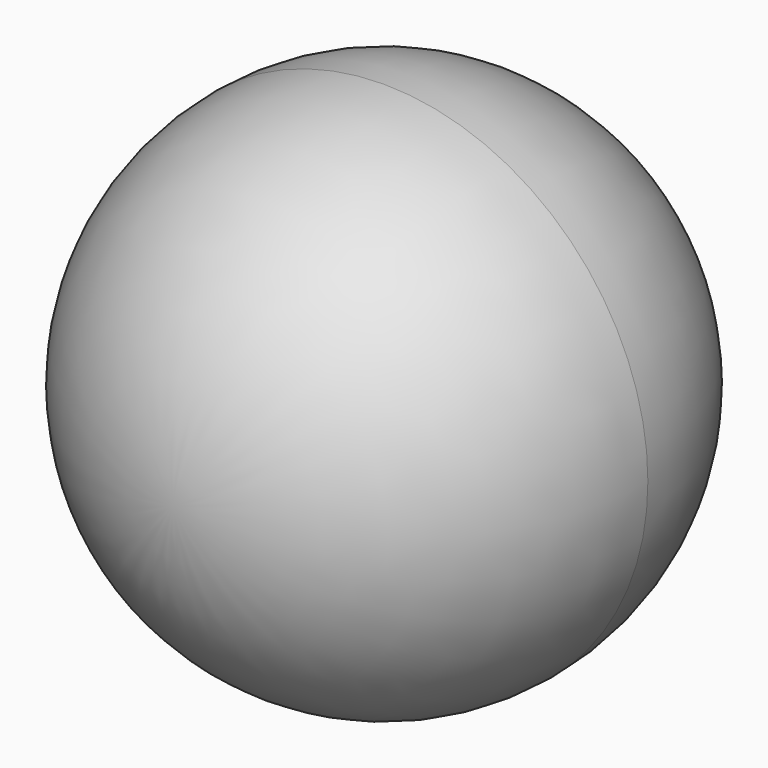
from build123d import *

# Parameters (mm, degrees)
F0_R     = 95.25
F1_DEPTH = 190.5
F2_R     = 95.24999


# Not quite as in the source:
# - a fillet or chamfer is up to 0.001 mm smaller than in the source, because OpenCascade refuses the exact size


with BuildPart() as f1:
    # F0 (on Front) → F1 (new body)
    with BuildSketch(Plane.XZ):
        Circle(F0_R)
    extrude(amount=F1_DEPTH)

    # F2 (radius 95.25 in the source; OpenCascade refuses exactly that, so slightly less here)
    f2_edges = [f1.edges().sort_by_distance(p)[0] for p in [
        (-95.25, -190.5, 0),
        (-95.25, 0, 0),
    ]]
    fillet(f2_edges, radius=F2_R)


solid = f1.part
